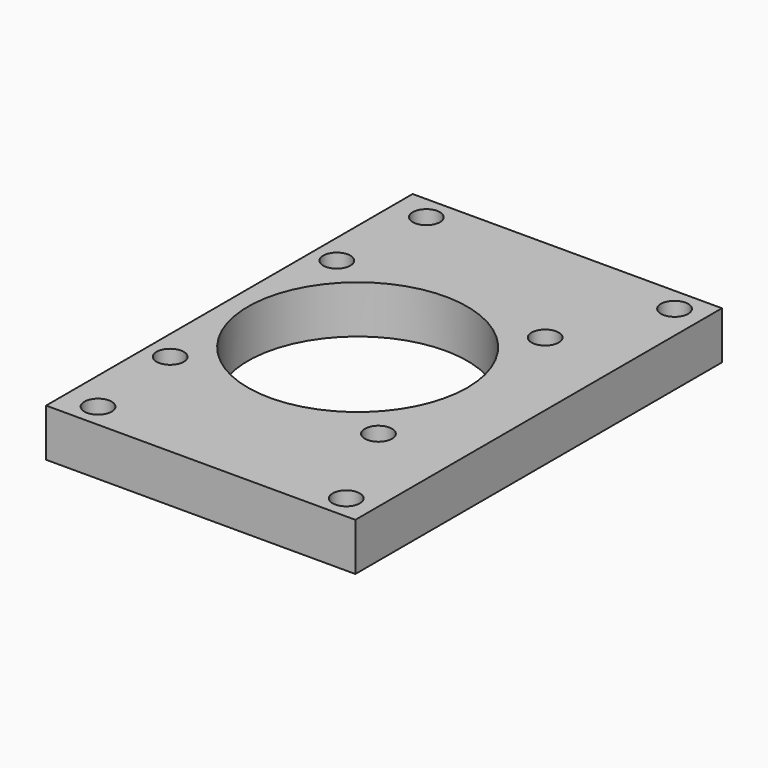
from build123d import *

# Parameters (mm, degrees)
F0_W     = 102.87
F0_H     = 152.4
F0_R     = 4.5212
F1_DEPTH = 15.875
F2_DEPTH = 197
F3_R     = 36.4998
F4_DEPTH = 15.876
F5_R     = 4.5212
F6_DEPTH = 15.876


# Not quite as in the source:
# - an extrude ends at something that could not be found from the text; its depth is read off the source's solid


with BuildPart() as f1:
    # F0 (on Top) → F1 (new body)
    with BuildSketch(Plane.XY):
        with Locations((8.763, 0)):
            Rectangle(F0_W, F0_H)
        with Locations((-31.75, -68.2498)):
            Circle(F0_R, mode=Mode.SUBTRACT)
        with Locations((50.8, -68.2498)):
            Circle(F0_R, mode=Mode.SUBTRACT)
        with Locations((-31.75, 68.2498)):
            Circle(F0_R, mode=Mode.SUBTRACT)
        with Locations((50.8, 68.2498)):
            Circle(F0_R, mode=Mode.SUBTRACT)
    extrude(amount=F1_DEPTH)

    # F0 (on Top) → F2 (cut, through all)
    with BuildSketch(Plane.XY):
        with Locations((8.763, 0)):
            Rectangle(F0_W, F0_H)
        with Locations((-31.75, -68.2498)):
            Circle(F0_R, mode=Mode.SUBTRACT)
        with Locations((50.8, -68.2498)):
            Circle(F0_R, mode=Mode.SUBTRACT)
        with Locations((-31.75, 68.2498)):
            Circle(F0_R, mode=Mode.SUBTRACT)
        with Locations((50.8, 68.2498)):
            Circle(F0_R, mode=Mode.SUBTRACT)
    extrude(amount=-F2_DEPTH, mode=Mode.SUBTRACT)

    # F3 (on face) → F4 (cut, through all)
    with BuildSketch(Plane.XY.offset(15.875)):
        Circle(F3_R)
    extrude(amount=-F4_DEPTH, mode=Mode.SUBTRACT)

    # F5 (on face) → F6 (cut, through all)
    with BuildSketch(Plane.XY.offset(15.875)):
        with Locations((-34.6456, 34.6456)):
            Circle(F5_R)
        with Locations((34.6456, 34.6456)):
            Circle(F5_R)
        with Locations((34.6456, -34.6456)):
            Circle(F5_R)
        with Locations((-34.6456, -34.6456)):
            Circle(F5_R)
    extrude(amount=-F6_DEPTH, mode=Mode.SUBTRACT)


solid = f1.part
